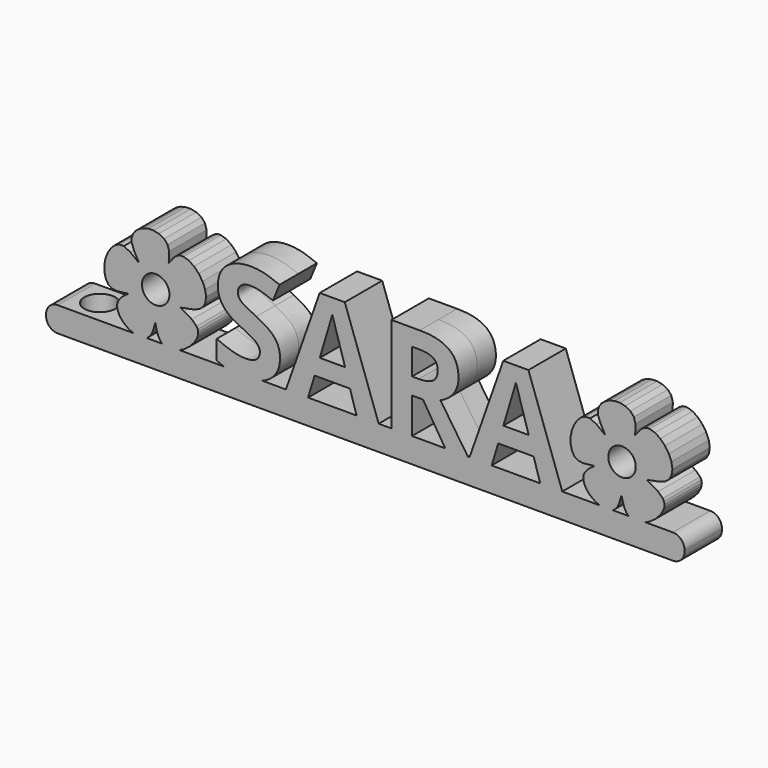
from build123d import *

# Parameters (mm, degrees)
F0_R         = 1.7660260944
F0_TEXT_SIZE = 17.4656599654
F1_DEPTH     = 3
F2_W         = 74.5
F2_H         = 6
F3_DEPTH     = 0.2
F4_DEPTH     = 3
F5_W         = 6
F5_H         = 3.2
F6_DEPTH     = 7.5
F7_R         = 1.5
F8_R         = 2
F9_DEPTH     = 4
F10_R        = 1.5


# Not quite as in the source:
# - Text() gives the source's letters only with a copy of the font that has no kerning and outlines rounded to 1/6400 em; it was checked with that copy


with BuildPart() as f1:
    # F0 (on Front) → F1 (new body, symmetric)
    with BuildSketch(Plane.XZ):
        Polygon((-9.8962181259, -0.0299609487), (-9.3093152472, 0.0995427735), (-8.5310452338, 0.4643787281), (-7.7886221935, 1.0156229815), (-7.1753136859, 1.6703047867), (-6.7844076966, 2.345448762), (-6.6844409889, 2.697736103), (-6.6652413988, 3.0240118702), (-6.7312263226, 3.3305926174), (-6.8868132072, 3.6238062576), (-7.4844896445, 4.1953846804), (-8.4936258745, 4.789299945), (-8.9274018823, 5.0567831788), (-8.4181052429, 5.1580766137), (-7.3131137554, 5.3695361907), (-6.5480905692, 5.6521941874), (-6.0523445823, 6.043851435), (-5.7552051187, 6.5823041299), (-5.6420905942, 7.3346827833), (-5.7751165223, 8.1369112107), (-6.1089634595, 8.9328581362), (-6.5983028952, 9.6663968681), (-7.1978267956, 10.281407439), (-7.8622157172, 10.7217585729), (-8.546147975, 10.9313258196), (-8.8812811082, 10.9320270148), (-9.2043064176, 10.8539824368), (-9.6469000392, 10.5612860557), (-10.1400767255, 9.9810366231), (-10.4508130024, 9.5801644376), (-10.4068223535, 10.0271686751), (-10.3916193646, 10.9311557532), (-10.598433195, 11.6324207168), (-11.0363252865, 12.1480644274), (-11.7143548393, 12.4951945719), (-12.3982545289, 12.6383143795), (-13.0712303381, 12.6247535348), (-13.7032208938, 12.4733707309), (-14.2641853, 12.2030313855), (-14.7240621838, 11.8325941916), (-15.0528129411, 11.3809291004), (-15.2203761991, 10.8668948051), (-15.1967042361, 10.3093544817), (-14.8286469794, 9.4077545862), (-14.3529716358, 8.5454741101), (-14.2906102139, 8.4004774316), (-14.4811582303, 8.5293860258), (-15.3946726039, 9.2300894295), (-16.21802192, 9.6332437342), (-16.8030362894, 9.634121823), (-17.3568401554, 9.3699870508), (-17.8525159958, 8.8932532172), (-18.2631576982, 8.2563454299), (-18.5618432066, 7.5116797807), (-18.7216618753, 6.7116836696), (-18.7156984739, 5.9087754295), (-18.5170445979, 5.1553756349), (-18.2008868091, 4.6439944488), (-17.7512302174, 4.3560670179), (-17.1086136552, 4.2712956407), (-16.2135760559, 4.3694053341), (-15.7044514474, 4.4302814773), (-15.6696932647, 4.4000047008), (-15.7790195709, 4.3290260096), (-16.1651405309, 4.0708069691), (-16.5523139664, 3.7127982689), (-16.8671052824, 3.3322639471), (-17.0360798838, 3.0064680418), (-17.0831036318, 2.6043628391), (-17.0239245605, 2.1921008316), (-16.867618816, 1.7819255621), (-16.6232807801, 1.3860941234), (-16.3000002503, 1.0168545414), (-15.9068693162, 0.6864593752), (-15.4529754831, 0.4071521172), (-14.9474063577, 0.1911989779), (-14.4397479673, 0.0570083052), (-13.9840845603, 0.0188926715), (-13.5797273957, 0.0772799851), (-13.2259605822, 0.2326232662), (-12.9220907946, 0.485341356), (-12.6674066752, 0.8358849825), (-12.4612081239, 1.2846821047), (-12.3027905578, 1.8321743328), (-12.1879723822, 2.2557758958), (-12.1309056827, 2.0998483864), (-12.0112204133, 1.5291342486), (-11.8237778137, 0.9902805659), (-11.5954117235, 0.5466869075), (-11.3529559319, 0.2617414835), (-10.9521058183, 0.053843468), (-10.4551700276, -0.0442881949), align=None)
        with Locations((-12.1185852993, 6.0541479067)):
            Circle(F0_R, mode=Mode.SUBTRACT)
        Polygon((49.7433384922, 9.9810366231), (49.4326022154, 9.5801644376), (49.4765928642, 10.0271686751), (49.4917958531, 10.9311557532), (49.2849820227, 11.6324207168), (48.8470899313, 12.1480644274), (48.1690603785, 12.4951945719), (47.4851606888, 12.6383143795), (46.8121848797, 12.6247535348), (46.180194324, 12.4733707309), (45.6192299178, 12.2030313855), (45.159353034, 11.8325941916), (44.8306022766, 11.3809291004), (44.6630390186, 10.8668948051), (44.6867109816, 10.3093544817), (45.0547682383, 9.4077545862), (45.5304435819, 8.5454741101), (45.5928050038, 8.4004774316), (45.4022569875, 8.5293860258), (44.4887426139, 9.2300894295), (43.6653932978, 9.6332437342), (43.0803789284, 9.634121823), (42.5265750624, 9.3699870508), (42.0308992219, 8.8932532172), (41.6202575196, 8.2563454299), (41.3215720111, 7.5116797807), (41.1617533425, 6.7116836696), (41.1677167439, 5.9087754295), (41.3663706199, 5.1553756349), (41.6825284087, 4.6439944488), (42.1321850004, 4.3560670179), (42.7748015626, 4.2712956407), (43.6698391619, 4.3694053341), (44.1789637704, 4.4302814773), (44.2137219531, 4.4000047008), (44.1043956469, 4.3290260096), (43.7182746869, 4.0708069691), (43.3311012514, 3.7127982689), (43.0163099354, 3.3322639471), (42.847335334, 3.0064680418), (42.8003115859, 2.6043628391), (42.8594906573, 2.1921008316), (43.0157964017, 1.7819255621), (43.2601344376, 1.3860941234), (43.5834149674, 1.0168545414), (43.9765459016, 0.6864593752), (44.4304397347, 0.4071521172), (44.9360088601, 0.1911989779), (45.4436672504, 0.0570083052), (45.8993306575, 0.0188926715), (46.303687822, 0.0772799851), (46.6574546356, 0.2326232662), (46.9613244231, 0.485341356), (47.2160085425, 0.8358849825), (47.4222070939, 1.2846821047), (47.58062466, 1.8321743328), (47.6954428355, 2.2557758958), (47.752509535, 2.0998483864), (47.8721948044, 1.5291342486), (48.059637404, 0.9902805659), (48.2880034942, 0.5466869075), (48.5304592859, 0.2617414835), (48.9313093995, 0.053843468), (49.4282451902, -0.0442881949), (49.9871970919, -0.0299609487), (50.5740999706, 0.0995427735), (51.352369984, 0.4643787281), (52.0947930243, 1.0156229815), (52.7081015319, 1.6703047867), (53.0990075212, 2.345448762), (53.1989742289, 2.697736103), (53.2181738189, 3.0240118702), (53.1521888951, 3.3305926174), (52.9966020106, 3.6238062576), (52.3989255733, 4.1953846804), (51.3897893432, 4.789299945), (50.9560133355, 5.0567831788), (51.4653099749, 5.1580766137), (52.5703014624, 5.3695361907), (53.3353246485, 5.6521941874), (53.8310706354, 6.043851435), (54.128210099, 6.5823041299), (54.2413246235, 7.3346827833), (54.1082986954, 8.1369112107), (53.7744517583, 8.9328581362), (53.2851123226, 9.6663968681), (52.6855884222, 10.281407439), (52.0211995006, 10.7217585729), (51.3372672428, 10.9313258196), (51.0021341095, 10.9320270148), (50.6791088002, 10.8539824368), (50.2365151785, 10.5612860557), align=None)
        with Locations((47.7648299184, 6.0541479067)):
            Circle(F0_R, mode=Mode.SUBTRACT)
        with Locations((-5.0849722551, 0)):
            Text('SARA', F0_TEXT_SIZE, font='Open Sans', font_style=FontStyle.BOLD, text_align=(TextAlign.LEFT, TextAlign.BOTTOM))
    extrude(amount=F1_DEPTH, both=True)



with BuildPart() as f3:
    # F2 (on Top) → F3 (new body)
    with BuildSketch(Plane.XY):
        with Locations((18.55, 0)):
            Rectangle(F2_W, F2_H)
    extrude(amount=F3_DEPTH)


with BuildPart() as f4:
    # F4 (new): a face of the model
    f4_faces = [f3.part.faces().sort_by_distance(p)[0] for p in [
        (18.55, 0, 0),
    ]]
    extrude(f4_faces, amount=F4_DEPTH)


with BuildPart() as f1_1:
    add(f1.part)

    add(f3.part)  # F6 merges F3

    add(f4.part)  # F6 merges F4
    # F5 (on face) → F6 (join)
    with BuildSketch(Plane(origin=(-18.7, 0, 0), x_dir=(0, -1, 0), z_dir=(-1, 0, 0))):
        with Locations((0, -1.4)):
            Rectangle(F5_W, F5_H)
    extrude(amount=F6_DEPTH)

    # F7
    f7_edges = [f1_1.edges().sort_by_distance(p)[0] for p in [
        (-26.2, 0, -3),
        (-26.2, 0, 0.2),
        (55.8, 0, -3),
    ]]
    fillet(f7_edges, radius=F7_R)

    # F8 (on face) → F9 (cut)
    with BuildSketch(Plane.XY.offset(0.2)):
        with Locations((-21.7, 0)):
            Circle(F8_R)
    extrude(amount=-F9_DEPTH, mode=Mode.SUBTRACT)

    # F10
    f10_edges = [f1_1.edges().sort_by_distance(p)[0] for p in [
        (55.8, 0, 0.2),
    ]]
    fillet(f10_edges, radius=F10_R)


solid = f1_1.part
